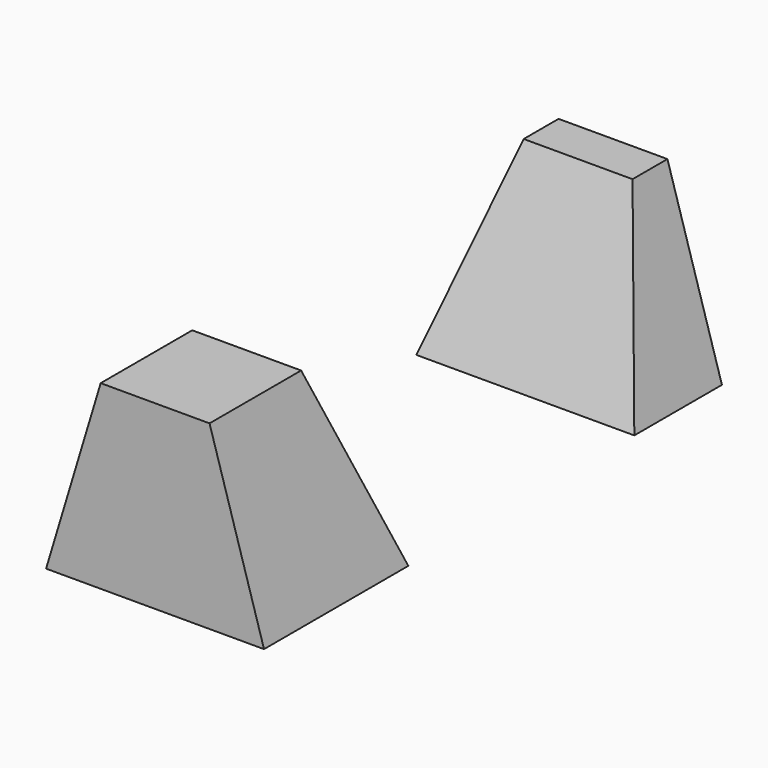
from build123d import *

# Parameters (mm, degrees)
F1_DEPTH    = 23.368
F2_T1_DEPTH = 285.3238303429
F4_DEPTH    = 6.604


# Not quite as in the source:
# - a fillet or chamfer that OpenCascade refuses, or shapes differently, is made with other operations: its cross-section is extruded or revolved along the edge and cut away or added


with BuildPart() as f1:
    # F0 (on Front) → F1 (new body)
    with BuildSketch(Plane.XZ):
        Polygon((0, -8.3422744647), (0, 0), (0, 8.5318721831), (-5.0714211538, 8.5318721831), (-10.1590277627, -8.3422744647), align=None)
        Polygon((0, 8.5318721831), (0, 0), (0, -8.3422744647), (10.1518854499, -8.3422744647), (5.0742193125, 8.5318721831), align=None)
    extrude(amount=F1_DEPTH)

    # F2: chamfer of 19.304 x 53.0373041052 on 1 edges, made by hand

    # F2_s2 → F2_t1 (cut)
    with BuildSketch(Plane.YZ.offset(-142.6605160921)):
        Polygon((-19.304, 8.5318721831), (0, -44.5054319221), (0, 8.5318721831), align=None)
    extrude(amount=F2_T1_DEPTH, mode=Mode.SUBTRACT)


with BuildPart() as f3_1:
    # F3: instance of F1
    add(f1.part.mirror(Plane.XZ))


with BuildPart() as f1_1:
    add(f1.part)

    # F4 (add): a face of the model
    f4_faces = [f1_1.faces().sort_by_distance(p)[0] for p in [
        (-0.0013625187, -23.368, -0.8438622953),
    ]]
    extrude(f4_faces, amount=F4_DEPTH)


solid = Compound([f3_1.part, f1_1.part])
